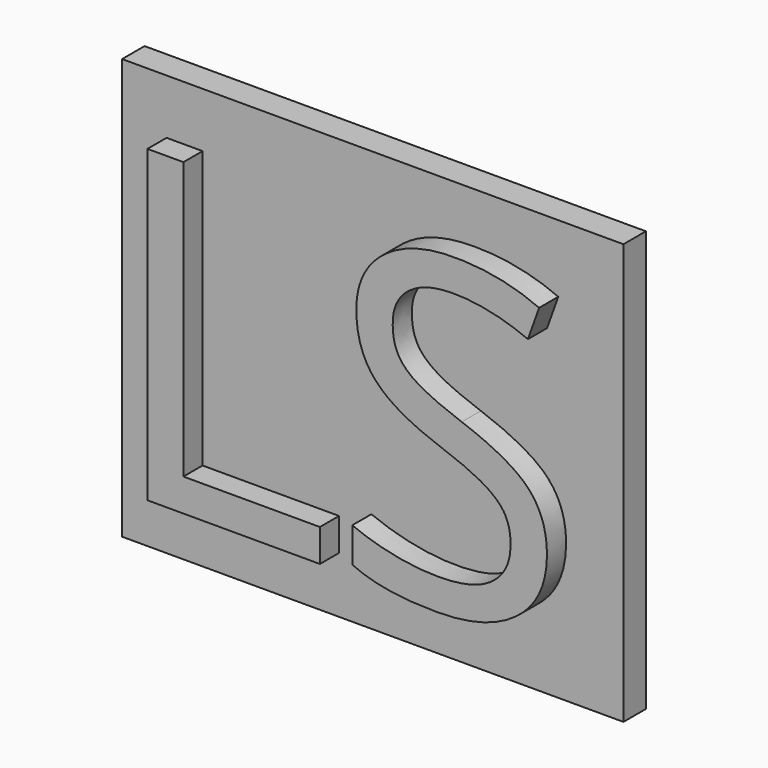
from build123d import *

# Parameters (mm, degrees)
F0_TEXT_SIZE = 105.8333333333
F1_DEPTH     = 12.7
F3_W         = 122.4374696612
F3_H         = 102.70376876
F4_DEPTH     = 6.858


# Not quite as in the source:
# - Text() gives the source's letters only with a copy of the font that has no kerning and outlines rounded to 1/6400 em; it was checked with that copy


with BuildPart() as f1:
    # F0 (on Front) → F1 (new body)
    with BuildSketch(Plane.XZ):
        with Locations((-51.6860431411, -37.6569770491)):
            Text('LS', F0_TEXT_SIZE, font='Open Sans', text_align=(TextAlign.LEFT, TextAlign.BOTTOM))
    extrude(amount=F1_DEPTH)

    # F3 (on face) → F4 (join)
    with BuildSketch(Plane.XZ):
        with Locations((9.0526156127, -0.0517945737)):
            Rectangle(F3_W, F3_H)
    extrude(amount=F4_DEPTH)


solid = f1.part
